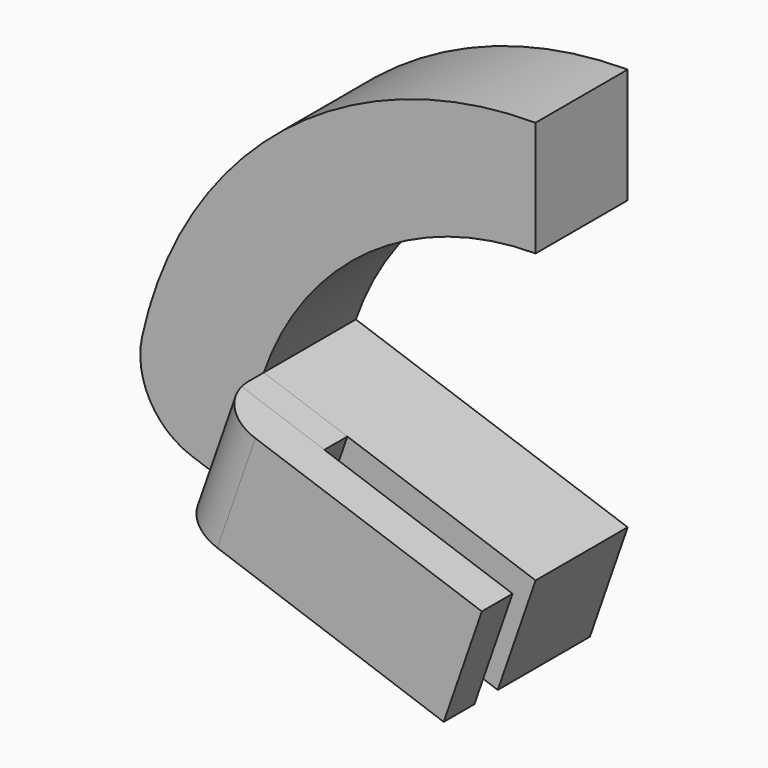
from build123d import *

# Parameters (mm, degrees)
F0_R        = 1.5
F1_DEPTH    = 6
F3_DEPTH    = 3
F5_DEPTH    = 4
F6_R        = 8
F7_T1_DEPTH = 37.0000029882


# Not quite as in the source:
# - a fillet or chamfer that OpenCascade refuses, or shapes differently, is made with other operations: its cross-section is extruded or revolved along the edge and cut away or added


with BuildPart() as f1:
    # F0 (on Front) → F1 (new body, symmetric)
    with BuildSketch(Plane.XZ):
        with BuildLine():
            ThreePointArc((-28.3348189516, 9.855862975), (-17.3828091911, 24.4507248282), (0, 30))
            Line((0, 30), (0, 42))
            ThreePointArc((0, 42), (-29.0229029625, 30.3590366057), (-41.9574939735, 1.8891001728))
            Line((-41.9574939735, 1.8891001728), (-3.94234519, -11.3339275806))
            Line((-3.94234519, -11.3339275806), (0, 0))
            Line((0, 0), (-28.3348189516, 9.855862975))
        make_face()
        with Locations((-5, -4.5450530015)):
            Circle(F0_R, mode=Mode.SUBTRACT)
    extrude(amount=F1_DEPTH, both=True)

    # F2 (on face) → F3 (join)
    with BuildSketch(Plane.XZ.offset(6)):
        Polygon((-19.6181767132, 6.8239031926), (-28.3348189516, 9.855862975), (-32.2851626761, -1.4752824294), (-23.5605219032, -4.5100243881), align=None)
    extrude(amount=F3_DEPTH)

    # F4 (on face) → F5 (join)
    with BuildSketch(Plane.XZ.offset(9)):
        Polygon((0, 0), (-28.3348189516, 9.855862975), (-32.2851626761, -1.4752824294), (-3.9770946697, -11.4338295597), align=None)
    extrude(amount=F5_DEPTH)

    # F6
    f6_edges = [f1.edges().sort_by_distance(p)[0] for p in [
        (-41.957494, 0, 1.8891),
    ]]
    fillet(f6_edges, radius=F6_R)

    # F7: fillet of radius 5 on 1 edges, made by hand

    # F7_s2 → F7_t1 (cut)
    with BuildSketch(Plane(origin=(4.1079708061, 0, 11.783282106), x_dir=(0, 1, 0), z_dir=(-0.3291952284, 0, -0.9442618819))):
        with BuildLine():
            ThreePointArc((-8, -29.9999925295), (-11.5355339059, -28.5355264354), (-13, -24.9999925295))
            Line((-13, -24.9999925295), (-13, -29.9999925295))
            Line((-13, -29.9999925295), (-8, -29.9999925295))
        make_face()
    extrude(amount=F7_T1_DEPTH, mode=Mode.SUBTRACT)


solid = f1.part
